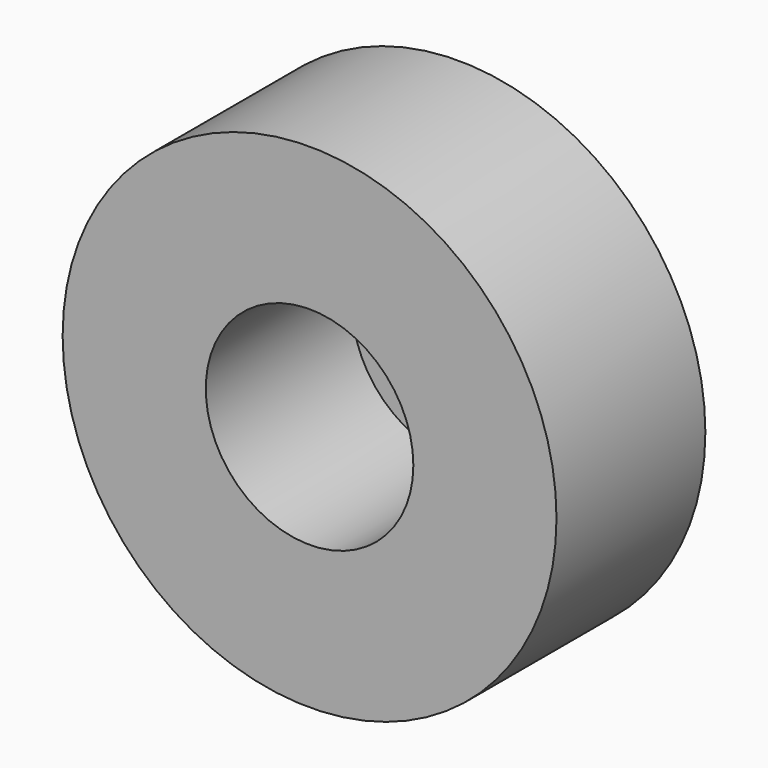
from build123d import *

# Parameters (mm, degrees)
F0_R     = 17.526
F1_DEPTH = 13.208
F2_R     = 7.366
F3_DEPTH = 12.9794


# Not quite as in the source:
# - a feature names something its author has since deleted; it is built from what else it names


with BuildPart() as f1:
    # F0 (on Front) → F1 (new body)
    with BuildSketch(Plane.XZ):
        Circle(F0_R)
    extrude(amount=F1_DEPTH)

    # F2 (on face) → F3 (cut)
    with BuildSketch(Plane.XZ.offset(13.208)):
        Circle(F2_R)
    extrude(amount=-F3_DEPTH, mode=Mode.SUBTRACT)


solid = f1.part
